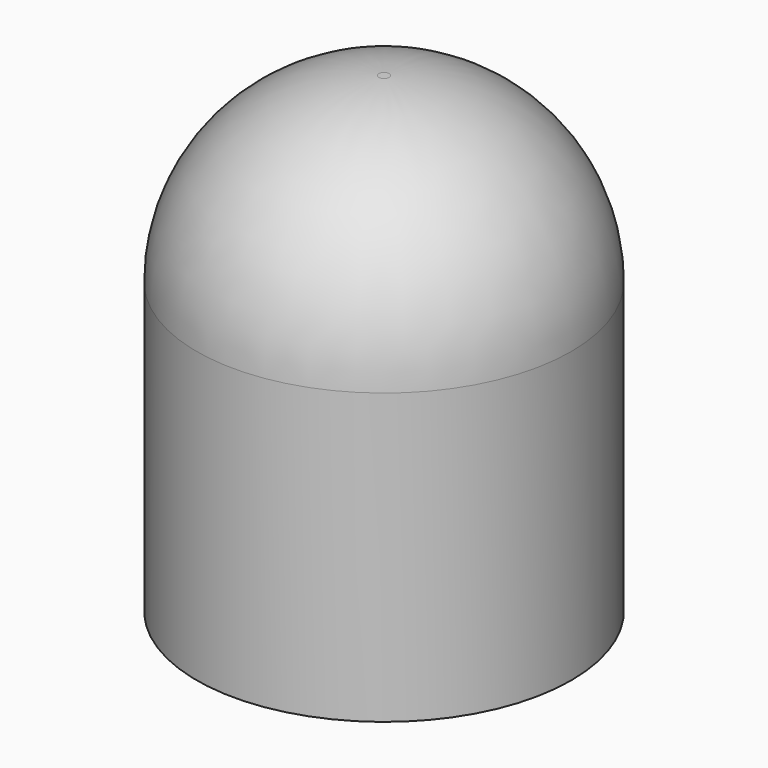
from build123d import *

# Parameters (mm, degrees)
F0_R     = 7.15
F0_R_2   = 6.75
F1_DEPTH = 18
F2_R     = 6.95
F3_T     = -0.42


with BuildPart() as f1:
    # F0 (on Top) → F1 (new body)
    with BuildSketch(Plane.XY):
        Circle(F0_R)
        Circle(F0_R_2, mode=Mode.SUBTRACT)
        Circle(F0_R_2)
    extrude(amount=F1_DEPTH)

    # F2
    f2_edges = [f1.edges().sort_by_distance(p)[0] for p in [
        (-7.15, 0, 18),
    ]]
    fillet(f2_edges, radius=F2_R)

    # F3
    f3_openings = [f1.faces().sort_by_distance(p)[0] for p in [
        (0, 0, 0),
    ]]
    offset(amount=F3_T, openings=f3_openings)


solid = f1.part
